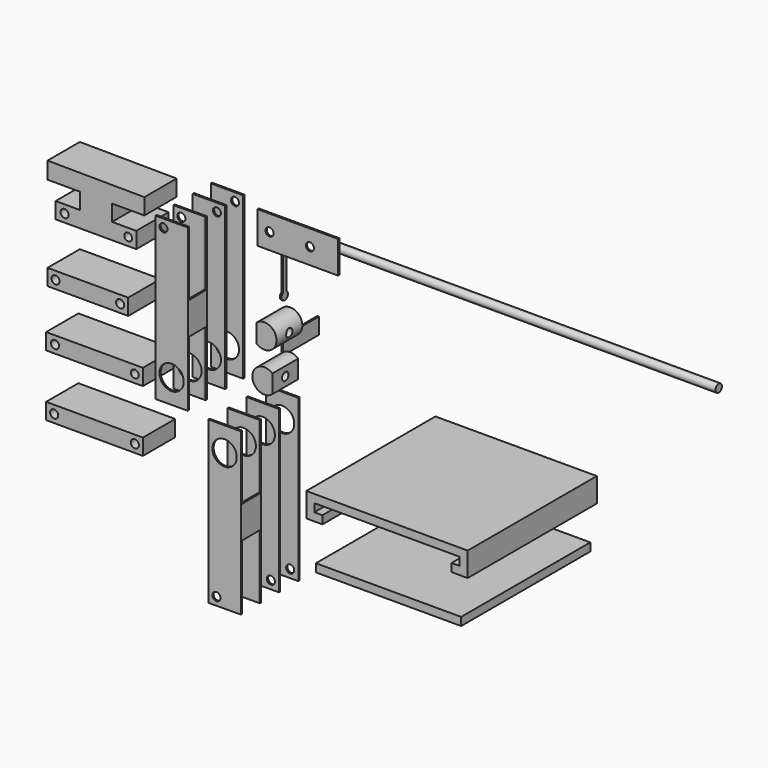
from build123d import *

# Parameters (mm, degrees)
F1_DEPTH  = 100
F2_R      = 7.5
F2_R_2    = 2.5
F3_DEPTH  = 15.001
F4_W      = 13
F4_H      = 40
F5_DEPTH  = 20.1627097718
F6_DEPTH  = 100
F7_R      = 7.5
F7_R_2    = 2.5
F8_DEPTH  = 16.001
F9_W      = 14
F9_H      = 40
F10_DEPTH = 20.1691592966
F11_W     = 50
F11_H     = 20
F11_R     = 2.5
F12_DEPTH = 1
F13_R     = 2.5
F13_R_2   = 7.5
F14_DEPTH = 45.1330833913
F15_R     = 7.5
F15_R_2   = 2.5
F16_DEPTH = 46.1330833913
F17_W     = 14
F17_H     = 40
F18_DEPTH = 53.5847666336
F19_W     = 13
F19_H     = 40
F20_DEPTH = 25
F22_DEPTH = 20
F23_R     = 2.5
F24_DEPTH = 250
F25_W     = 50
F25_H     = 10
F25_R     = 2.5
F26_DEPTH = 25
F25_R_2   = 2.4144593705
F25_W_2   = 60
F27_DEPTH = 25
F28_R     = 2.5
F29_DEPTH = 136.2251037518
F30_R     = 2.5
F31_DEPTH = 214.5146418358
F33_DEPTH = 1
F34_W     = 1
F34_H     = 10
F35_DEPTH = 25
F37_DEPTH = 100


# Not quite as in the source:
# - a feature names something its author has since deleted; it is built from what else it names


with BuildPart() as f1:
    # F0 (on Top) → F1 (new body)
    with BuildSketch(Plane.XY):
        Polygon((0, 14), (0, 15), (-20, 15), (-20, 0), (0, 0), (0, 1), (-19, 1), (-19, 14), align=None)
    extrude(amount=F1_DEPTH)

    # F2 (on face) → F3 (cut, through all)
    with BuildSketch(Plane.XZ):
        with Locations((-10, 15)):
            Circle(F2_R)
        with Locations((-5, 95)):
            Circle(F2_R_2)
    extrude(amount=-F3_DEPTH, mode=Mode.SUBTRACT)

    # F4 (on face) → F5 (cut, through all)
    with BuildSketch(Plane(origin=(-20, 0, 0), x_dir=(0, -1, 0), z_dir=(-1, 0, 0))):
        with Locations((-7.5, 20)):
            Rectangle(F4_W, F4_H)
        with Locations((-7.5, 80)):
            Rectangle(F4_W, F4_H)
    extrude(amount=-F5_DEPTH, mode=Mode.SUBTRACT)


with BuildPart() as f1b:
    # F0 (on Top) → F1, piece 2 (new body)
    with BuildSketch(Plane.XY):
        Polygon((0.051417134, -13.985459061), (-19.9480422158, -14.1325159114), (-19.9406893732, -15.1324888789), (-0.941202991, -14.992784871), (-0.8456160382, -27.9924334484), (-19.837749578, -28.1320833905), (-19.837749578, -29.1321104238), (0.1617097718, -28.9850535734), align=None)
    extrude(amount=F1_DEPTH)

    # F13 (on face) → F14 (cut, through all)
    with BuildSketch(Plane(origin=(0.2131255159, -28.9846755113, 0), x_dir=(0.9999729675, 0.0073528425, 0), z_dir=(0.0073528425, -0.9999729675, 0))):
        with Locations((-15.051417134, 95)):
            Circle(F13_R)
        with Locations((-10.051417134, 15)):
            Circle(F13_R_2)
    extrude(amount=-F14_DEPTH, mode=Mode.SUBTRACT)

    # F19 (on face) → F20 (cut)
    with BuildSketch(Plane(origin=(-0.0514157441, -0.0003780621, 0), x_dir=(-0.0073528425, 0.9999729675, 0), z_dir=(0.9999729675, 0.0073528425, 0))):
        with Locations((-21.485459061, 20)):
            Rectangle(F19_W, F19_H)
        with Locations((-21.485459061, 80)):
            Rectangle(F19_W, F19_H)
    extrude(amount=-F20_DEPTH, mode=Mode.SUBTRACT)


with BuildPart() as f6:
    # F0 (on Top) → F6 (new body)
    with BuildSketch(Plane.XY):
        Polygon((33.4159745649, 0), (33.4159745649, 1), (14.4159745649, 1), (14.4159745649, 15), (33.4159745649, 15), (33.4159745649, 16), (13.4159745649, 16), (13.4159745649, 0), align=None)
    extrude(amount=-F6_DEPTH)

    # F7 (on face) → F8 (cut, through all)
    with BuildSketch(Plane.XZ):
        with Locations((23.4159745649, -15)):
            Circle(F7_R)
        with Locations((28.4159745649, -95)):
            Circle(F7_R_2)
    extrude(amount=-F8_DEPTH, mode=Mode.SUBTRACT)

    # F9 (on face) → F10 (cut, through all)
    with BuildSketch(Plane(origin=(13.4159745649, 0, 0), x_dir=(0, -1, 0), z_dir=(-1, 0, 0))):
        with Locations((-8, -20)):
            Rectangle(F9_W, F9_H)
        with Locations((-8, -80)):
            Rectangle(F9_W, F9_H)
    extrude(amount=-F10_DEPTH, mode=Mode.SUBTRACT)


with BuildPart() as f6b:
    # F0 (on Top) → F6, piece 2 (new body)
    with BuildSketch(Plane.XY):
        Polygon((33.4664883811, -13.7397566624), (13.4670290313, -13.8868135128), (13.4743818739, -14.8867864803), (32.4738682561, -14.7470824724), (32.5768080514, -28.7467040172), (13.5846745117, -28.8863539594), (13.5846745117, -29.8863809926), (33.5841338614, -29.7393241422), align=None)
    extrude(amount=-F6_DEPTH)

    # F15 (on face) → F16 (cut, through all)
    with BuildSketch(Plane(origin=(0.2204783584, -29.9846484788, 0), x_dir=(0.9999729675, 0.0073528425, 0), z_dir=(0.0073528425, -0.9999729675, 0))):
        with Locations((23.3645574309, -15)):
            Circle(F15_R)
        with Locations((18.3645574309, -95)):
            Circle(F15_R_2)
    extrude(amount=-F16_DEPTH, mode=Mode.SUBTRACT)

    # F17 (on face) → F18 (cut, through all)
    with BuildSketch(Plane(origin=(33.3636555031, 0.2453243365, 0), x_dir=(-0.0073528425, 0.9999729675, 0), z_dir=(0.9999729675, 0.0073528425, 0))):
        with Locations((-21.985459061, -20)):
            Rectangle(F17_W, F17_H)
        with Locations((-21.985459061, -80)):
            Rectangle(F17_W, F17_H)
    extrude(amount=-F18_DEPTH, mode=Mode.SUBTRACT)


with BuildPart() as f12:
    # F11 (on Front) → F12 (new body)
    with BuildSketch(Plane.XZ):
        with Locations((45.8931141218, 95.3558683395)):
            Rectangle(F11_W, F11_H)
        with Locations((28.3931141218, 95.3558683395)):
            Circle(F11_R, mode=Mode.SUBTRACT)
        with Locations((53.3931141218, 95.3558683395)):
            Circle(F11_R, mode=Mode.SUBTRACT)
    extrude(amount=F12_DEPTH)


with BuildPart() as f22:
    # F21 (on Front) → F22 (new body)
    with BuildSketch(Plane.XZ):
        with BuildLine():
            Line((35.4863581642, 55.8813297105), (35.4863581642, 44.6073331245))
            ThreePointArc((35.4863581642, 44.6073331245), (47.9335038306, 50.2443314175), (35.4863581642, 55.8813297105))
        make_face()
    extrude(amount=F22_DEPTH)

    # F30 (on face) → F31 (cut, through all)
    with BuildSketch(Plane(origin=(35.4863581642, 0, 0), x_dir=(0, -1, 0), z_dir=(-1, 0, 0))):
        with Locations((10, 50.2443314175)):
            Circle(F30_R)
    extrude(amount=-F31_DEPTH, mode=Mode.SUBTRACT)


with BuildPart() as f22b:
    # F21 (on Front) → F22, piece 2 (new body)
    with BuildSketch(Plane.XZ):
        with BuildLine():
            Line((45.380649497, 20.1312099156), (45.380649497, 31.4052065016))
            ThreePointArc((45.380649497, 31.4052065016), (32.9335038306, 25.7682082086), (45.380649497, 20.1312099156))
        make_face()
    extrude(amount=F22_DEPTH)

    # F28 (on face) → F29 (cut, through all)
    with BuildSketch(Plane.YZ.offset(45.380649497)):
        with Locations((-10, 25.7682082086)):
            Circle(F28_R)
    extrude(amount=-F29_DEPTH, mode=Mode.SUBTRACT)


with BuildPart() as f24:
    # F23 (on Right) → F24 (new body)
    with BuildSketch(Plane.YZ):
        with Locations((69.883659482, 53.4276850522)):
            Circle(F23_R)
    extrude(amount=F24_DEPTH)


with BuildPart() as f26:
    # F25 (on Front) → F26 (new body)
    with BuildSketch(Plane.XZ):
        with Locations((-64.9493469292, 42.0624911785)):
            Rectangle(F25_W, F25_H)
        with Locations((-84.9493469292, 42.0624911785)):
            Circle(F25_R, mode=Mode.SUBTRACT)
        with Locations((-44.9493469292, 42.0624911785)):
            Circle(F25_R, mode=Mode.SUBTRACT)
    extrude(amount=F26_DEPTH)


with BuildPart() as f26b:
    # F25 (on Front) → F26, piece 2 (new body)
    with BuildSketch(Plane.XZ):
        Polygon((-84.9493469292, 85.124527216), (-84.9493469292, 75.124527216), (-34.9493469292, 75.124527216), (-34.9493469292, 85.124527216), (-49.9493469292, 85.124527216), (-49.9493469292, 95.124527216), (-29.9493469292, 95.124527216), (-29.9493469292, 105.124527216), (-89.9493469292, 105.5638343096), (-89.9493469292, 95.124527216), (-69.9493469292, 95.124527216), (-69.9493469292, 85.124527216), align=None)
        with Locations((-79.3778774142, 80.124527216)):
            Circle(F25_R, mode=Mode.SUBTRACT)
        with Locations((-39.9493469292, 80.124527216)):
            Circle(F25_R_2, mode=Mode.SUBTRACT)
    extrude(amount=F26_DEPTH)


with BuildPart() as f27:
    # F25 (on Front) → F27 (new body)
    with BuildSketch(Plane.XZ):
        with Locations((-60.8434542548, -31.3186603598)):
            Rectangle(F25_W_2, F25_H)
        with Locations((-85.8434542548, -31.3186603598)):
            Circle(F25_R, mode=Mode.SUBTRACT)
        with Locations((-35.8434542548, -31.3186603598)):
            Circle(F25_R, mode=Mode.SUBTRACT)
    extrude(amount=F27_DEPTH)


with BuildPart() as f27b:
    # F25 (on Front) → F27, piece 2 (new body)
    with BuildSketch(Plane.XZ):
        with Locations((-60.8434542548, 6.7433756776)):
            Rectangle(F25_W_2, F25_H)
        with Locations((-85.2719847398, 6.7433756776)):
            Circle(F25_R, mode=Mode.SUBTRACT)
        with Locations((-35.8434542548, 6.7433756776)):
            Circle(F25_R_2, mode=Mode.SUBTRACT)
    extrude(amount=F27_DEPTH)


with BuildPart() as f33:
    # F32 (on Right) → F33 (new body)
    with BuildSketch(Plane.YZ):
        with BuildLine():
            Line((47.762863338, 8.6800148711), (47.762863338, 20.4667558931))
            ThreePointArc((47.762863338, 20.4667558931), (46.3052242994, 24.9978365004), (44.8475852609, 20.4667558931))
            Line((44.8475852609, 20.4667558931), (44.8475852609, 8.6800148711))
            Line((44.8475852609, 8.6800148711), (44.8475852609, 0))
            Line((44.8475852609, 0), (47.762863338, 0))
            Line((47.762863338, 0), (47.762863338, 8.6800148711))
        make_face()
    extrude(amount=-F33_DEPTH)

    # F34 (on face) → F35 (join)
    with BuildSketch(Plane(origin=(0, 47.762863338, 0), x_dir=(-1, 0, 0), z_dir=(0, 1, 0))):
        with Locations((0.5, 5)):
            Rectangle(F34_W, F34_H)
    extrude(amount=F35_DEPTH)


with BuildPart() as f33b:
    # F32 (on Right) → F33, piece 2 (new body)
    with BuildSketch(Plane.YZ):
        with BuildLine():
            ThreePointArc((44.8475852609, 34.1576339639), (46.3052242994, 29.6265533566), (47.762863338, 34.1576339639))
            Line((47.762863338, 34.1576339639), (47.762863338, 45.944374986))
            Line((47.762863338, 45.944374986), (47.762863338, 54.6243898571))
            Line((47.762863338, 54.6243898571), (44.8475852609, 54.6243898571))
            Line((44.8475852609, 54.6243898571), (44.8475852609, 45.944374986))
            Line((44.8475852609, 45.944374986), (44.8475852609, 34.1576339639))
        make_face()
    extrude(amount=-F33_DEPTH)


with BuildPart() as f37:
    # F36 (on Front) → F37 (new body)
    with BuildSketch(Plane.XZ):
        Polygon((220.3795283456, 17.4886658788), (220.3795283456, 12.4886658788), (230.3795283456, 12.4886658788), (230.3795283456, 27.4886658788), (180.3795283456, 27.4886658788), (130.3795283456, 27.4886658788), (130.3795283456, 12.4886658788), (140.3795283456, 12.4886658788), (140.3795283456, 17.4886658788), (135.3795283456, 17.4886658788), (135.3795283456, 22.4886658788), (180.3795283456, 22.4886658788), (225.3795283456, 22.4886658788), (225.3795283456, 17.4886658788), align=None)
    extrude(amount=F37_DEPTH)


with BuildPart() as f37b:
    # F36 (on Front) → F37, piece 2 (new body)
    with BuildSketch(Plane.XZ):
        Polygon((136.3347970862, -15.0014664978), (181.3347970862, -15.0014664978), (226.3347970862, -15.0014664978), (226.3347970862, -10.0014664978), (181.3347970862, -10.0014664978), (136.3347970862, -10.0014664978), align=None)
    extrude(amount=F37_DEPTH)


solid = Compound([f1.part, f1b.part, f6.part, f6b.part, f12.part, f22.part, f22b.part, f24.part, f26.part, f26b.part, f27.part, f27b.part, f33.part, f33b.part, f37.part, f37b.part])
